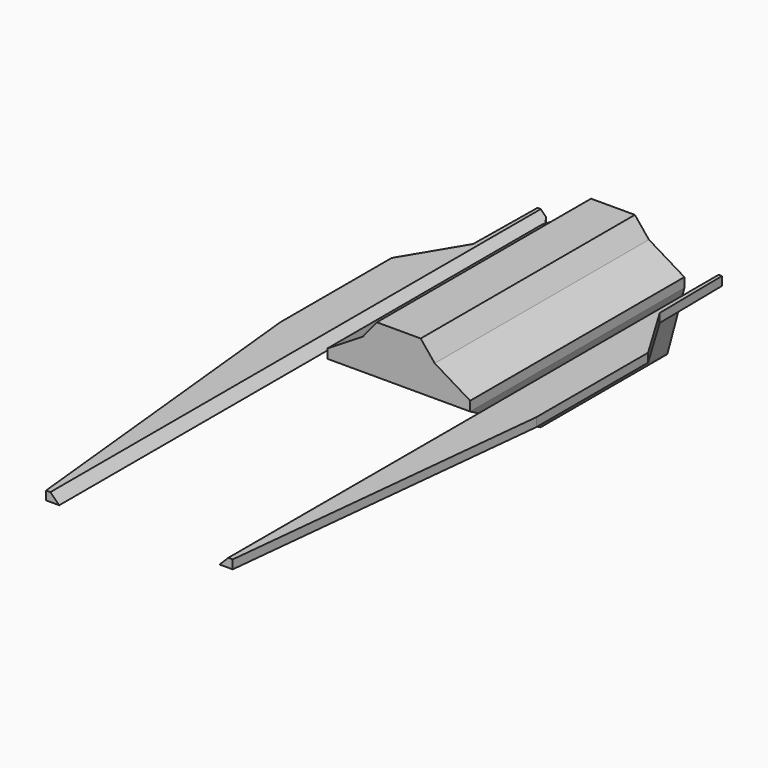
from build123d import *

# Parameters (mm, degrees)
F1_DEPTH       = 2.54
F2_W           = 41.3538680857
F2_H           = 77.5493303561
F3_DEPTH       = 19.05
F5_DEPTH       = 41.656
F6_SIZE2       = 19.05
F6_SIZE        = 5.08
F7_R           = 1.27
F9_DEPTH       = 83.595498357
F10_T1_DEPTH   = 197.5782991577
F10_2_T1_DEPTH = 197.5782991577


# Not quite as in the source:
# - a fillet or chamfer that OpenCascade refuses, or shapes differently, is made with other operations: its cross-section is extruded or revolved along the edge and cut away or added


with BuildPart() as f1:
    # F0 (on Top) → F1 (new body)
    with BuildSketch(Plane.XY):
        Polygon((-37.1346319619, 20.5705222299), (-27.0269340429, -76.7609926856), (-20.6769340429, -76.7609926856), (-20.6769340429, 94.6890073144), (-24.1763866916, 100.7341753154), (-26.7163866916, 100.7341753154), (-27.0269340429, 77.8327360749), (-37.1346319619, 60.9812401235), align=None)
    extrude(amount=F1_DEPTH)

    # F10#2: chamfer of 5.08 on 1 edges, made by hand

    # F10_2_s2 → F10_2_t1 (cut)
    with BuildSketch(Plane.XZ.offset(-107.7531568933)):
        Polygon((-20.6769340429, -2.54), (-25.7569340429, 2.54), (-20.6769340429, 2.54), align=None)
    extrude(amount=F10_2_T1_DEPTH, mode=Mode.SUBTRACT)


with BuildPart() as f1b:
    # F0 (on Top) → F1, piece 2 (new body)
    with BuildSketch(Plane.XY):
        Polygon((27.0269340429, 77.8327360749), (26.7163866916, 100.7341753154), (24.1763866916, 100.7341753154), (20.6769340429, 94.6890073144), (20.6769340429, -76.7609926856), (27.0269340429, -76.7609926856), (37.1346319619, 20.5705222299), (37.1346319619, 60.9812401235), align=None)
    extrude(amount=F1_DEPTH)

    # F10: chamfer of 5.08 on 1 edges, made by hand

    # F10_s2 → F10_t1 (cut)
    with BuildSketch(Plane.XZ.offset(-107.7531568933)):
        Polygon((20.6769340429, -2.54), (25.7569340429, 2.54), (20.6769340429, 2.54), align=None)
    extrude(amount=F10_T1_DEPTH, mode=Mode.SUBTRACT)


with BuildPart() as f3:
    # F2 (on Top) → F3 (new body, symmetric)
    with BuildSketch(Plane.XY):
        with Locations((0, 55.9143421364)):
            Rectangle(F2_W, F2_H)
    extrude(amount=F3_DEPTH, both=True)

    # F4 (on face) → F5 (cut)
    with BuildSketch(Plane.YZ.offset(20.6769340429)):
        Polygon((49.6939942241, -19.05), (17.1396769583, 0), (17.1396769583, -19.05), align=None)
    extrude(amount=-F5_DEPTH, mode=Mode.SUBTRACT)

    # F6
    f6_edges = [f3.edges().sort_by_distance(p)[0] for p in [
        (20.676934, 72.191501, -19.05),
        (-20.676934, 72.191501, -19.05),
    ]]
    f6_side = f3.faces().sort_by_distance((0, 72.191501, -19.05))[0]
    chamfer(f6_edges, length=F6_SIZE, length2=F6_SIZE2, reference=f6_side)

    # F7
    f7_edges = [f3.edges().sort_by_distance(p)[0] for p in [
        (15.596934, 72.191501, -19.05),
        (-15.596934, 72.191501, -19.05),
    ]]
    fillet(f7_edges, radius=F7_R)

    # F8 (on face) → F9 (cut, through all)
    with BuildSketch(Plane.XZ.offset(-17.1396769583)):
        Polygon((-20.6769340429, 19.05), (-20.6769340429, 2.6444371324), (-10.4151861742, 8.9688580483), (-6.3513340429, 13.97), (6.3486659571, 13.97), (10.4125180885, 8.9688580483), (20.6769340429, 2.762777498), (20.6769340429, 19.05), align=None)
    extrude(amount=-F9_DEPTH, mode=Mode.SUBTRACT)


solid = Compound([f1.part, f1b.part, f3.part])
